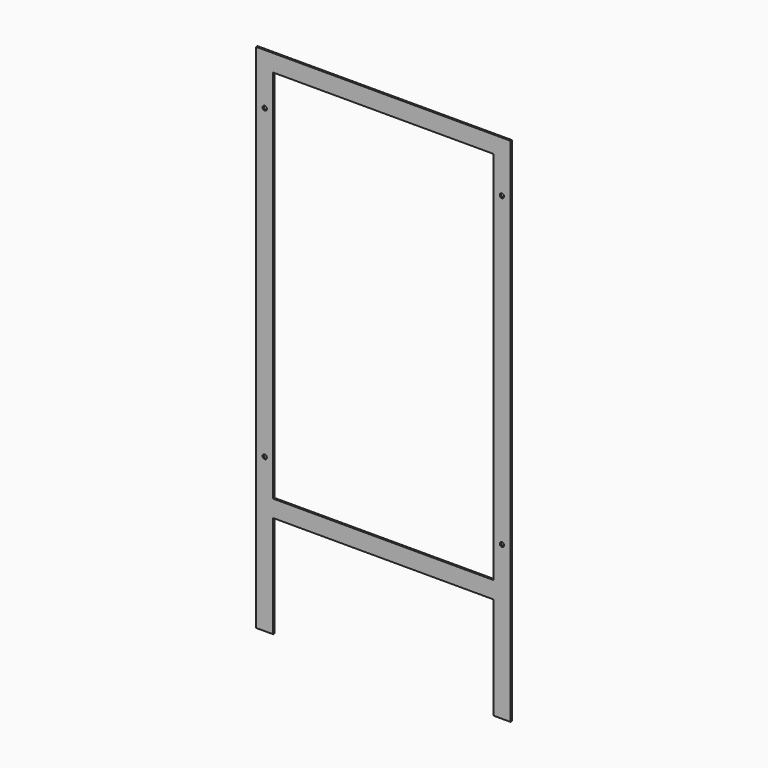
from build123d import *

# Parameters (mm, degrees)
F0_W     = 378.7394
F0_H     = 751.84
F0_H_2   = 10.16
F1_DEPTH = 2.54
F2_W     = 327.9394
F2_H     = 152.4
F2_H_2   = 558.8
F2_R     = 3.175
F3_DEPTH = 2.541


# Not quite as in the source:
# - a length typed as a fraction of an inch, garbled in the dataset ("3 / 203.2 mm" for 3/8 in), is restored


with BuildPart() as f1:
    # F0 (on Front) → F1 (new body)
    with BuildSketch(Plane.XZ):
        with Locations((0, -5.08)):
            Rectangle(F0_W, F0_H)
        with Locations((0, 375.92)):
            Rectangle(F0_W, F0_H_2)
    extrude(amount=F1_DEPTH)

    # F2 (on face) → F3 (cut, through all)
    with BuildSketch(Plane.XZ.offset(2.54)):
        with Locations((0, -304.8)):
            Rectangle(F2_W, F2_H)
        with Locations((0, 76.2)):
            Rectangle(F2_W, F2_H_2)
        with BuildLine():
            ThreePointArc((178.1250186398, 307.6218208052), (173.9584953156, 303.1477306033), (179.8447, 304.8))
            ThreePointArc((179.8447, 304.8), (179.3809046844, 306.4522693967), (178.1250186398, 307.6218208052))
        make_face()
        with BuildLine():
            ThreePointArc((176.6697, -149.225), (174.4246359697, -154.6450640303), (179.8447, -152.4))
            ThreePointArc((179.8447, -152.4), (178.9147640303, -150.1549359697), (176.6697, -149.225))
        make_face()
        with BuildLine():
            ThreePointArc((-176.6697, -149.225), (-178.9147640303, -154.6450640303), (-173.4947, -152.4))
            ThreePointArc((-173.4947, -152.4), (-174.4246359697, -150.1549359697), (-176.6697, -149.225))
        make_face()
        with Locations((-176.6697, 304.8)):
            Circle(F2_R)
    extrude(amount=-F3_DEPTH, mode=Mode.SUBTRACT)


solid = f1.part
